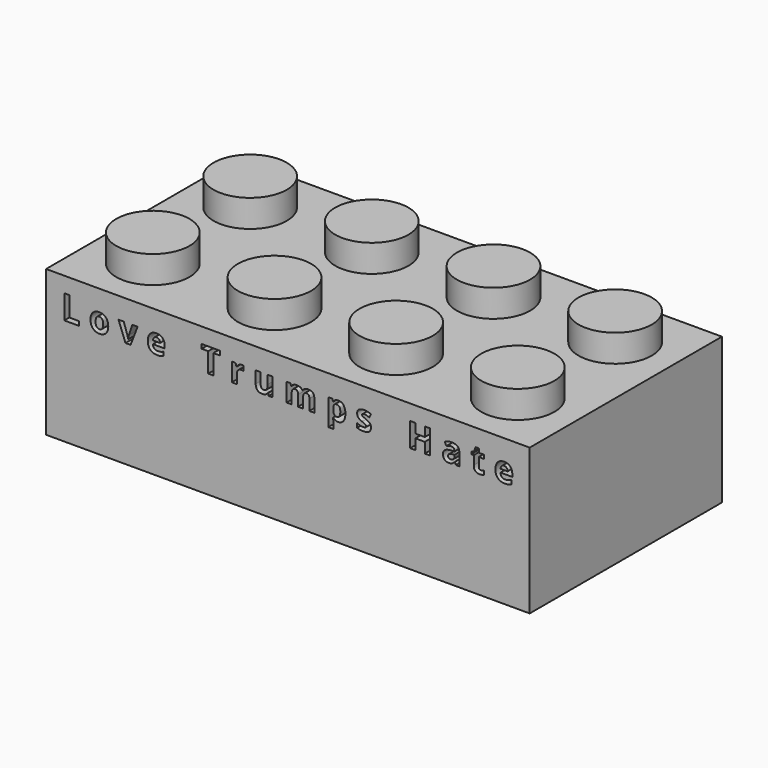
from build123d import *

# Parameters (mm, degrees)
F0_W          = 31.8
F0_H          = 15.8
F1_DEPTH      = 4.8
F2_W          = 29.4
F2_H          = 13.4
F3_DEPTH      = 8.6
F4_R          = 2.409
F5_DEPTH      = 1.8
F6_R          = 1.3
F7_DEPTH      = 1.2
F8_R          = 3.255
F8_R_2        = 2.4
F9_DEPTH      = 8.6
F10_W         = 0.3
F10_H         = 0.6
F11_DEPTH     = 8.6
F12_W         = 0.6
F12_H         = 0.3
F13_DEPTH     = 8.6
F14_W         = 0.8
F14_H         = 3.4696710694
F15_DEPTH     = 6.4
F16_TEXT_SIZE = 2.2075862628
F17_DEPTH     = 1


# Not quite as in the source:
# - Text() gives the source's letters only with a copy of the font that has no kerning and outlines rounded to 1/6400 em; it was checked with that copy


with BuildPart() as f1:
    # F0 (on Top) → F1 (new body, symmetric)
    with BuildSketch(Plane.XY):
        Rectangle(F0_W, F0_H)
    extrude(amount=F1_DEPTH, both=True)

    # F2 (on face) → F3 (cut)
    with BuildSketch(Plane(origin=(0, 0, -4.8), x_dir=(1, 0, 0), z_dir=(0, 0, -1))):
        Rectangle(F2_W, F2_H)
    extrude(amount=-F3_DEPTH, mode=Mode.SUBTRACT)

    # F4 (on face) → F5 (join)
    with BuildSketch(Plane.XY.offset(4.8)):
        with Locations((-12, 4)):
            Circle(F4_R)
        with Locations((-4, 4)):
            Circle(F4_R)
        with Locations((-12, -4)):
            Circle(F4_R)
        with Locations((-4, -4)):
            Circle(F4_R)
        with Locations((4, -4)):
            Circle(F4_R)
        with Locations((12, -4)):
            Circle(F4_R)
        with Locations((4, 4)):
            Circle(F4_R)
        with Locations((12, 4)):
            Circle(F4_R)
    extrude(amount=F5_DEPTH)

    # F6 (on face) → F7 (cut)
    with BuildSketch(Plane(origin=(0, 0, 3.8), x_dir=(1, 0, 0), z_dir=(0, 0, -1))):
        with Locations((-12, 4)):
            Circle(F6_R)
        with Locations((-4, 4)):
            Circle(F6_R)
        with Locations((-4, -4)):
            Circle(F6_R)
        with Locations((-12, -4)):
            Circle(F6_R)
        with Locations((4, -4)):
            Circle(F6_R)
        with Locations((12, -4)):
            Circle(F6_R)
        with Locations((4, 4)):
            Circle(F6_R)
        with Locations((12, 4)):
            Circle(F6_R)
    extrude(amount=-F7_DEPTH, mode=Mode.SUBTRACT)

    # F8 (on face) → F9 (join, through all)
    with BuildSketch(Plane(origin=(0, 0, 3.8), x_dir=(1, 0, 0), z_dir=(0, 0, -1))):
        with Locations((-8, 0)):
            Circle(F8_R)
        with Locations((-8, 0)):
            Circle(F8_R_2, mode=Mode.SUBTRACT)
        Circle(F8_R)
        Circle(F8_R_2, mode=Mode.SUBTRACT)
        with Locations((8, 0)):
            Circle(F8_R)
        with Locations((8, 0)):
            Circle(F8_R_2, mode=Mode.SUBTRACT)
    extrude(amount=F9_DEPTH)

    # F10 (on face) → F11 (join, through all)
    with BuildSketch(Plane(origin=(0, 0, 3.8), x_dir=(1, 0, 0), z_dir=(0, 0, -1))):
        Polygon((-14.7, 4.3), (-14.7, 3.7), (-14.4, 3.7), (-14.4, 4.2064064182), (-14.4, 4.2636040598), (-14.4, 4.3), align=None)
        with Locations((-14.55, -4)):
            Rectangle(F10_W, F10_H)
        with Locations((14.55, -4)):
            Rectangle(F10_W, F10_H)
        with Locations((14.55, 4)):
            Rectangle(F10_W, F10_H)
    extrude(amount=F11_DEPTH)

    # F12 (on face) → F13 (join, through all)
    with BuildSketch(Plane(origin=(0, 0, 3.8), x_dir=(1, 0, 0), z_dir=(0, 0, -1))):
        with Locations((-12, 6.55)):
            Rectangle(F12_W, F12_H)
        with Locations((-4, 6.55)):
            Rectangle(F12_W, F12_H)
        with Locations((4, 6.55)):
            Rectangle(F12_W, F12_H)
        with Locations((12, 6.55)):
            Rectangle(F12_W, F12_H)
        with Locations((-4, -6.55)):
            Rectangle(F12_W, F12_H)
        with Locations((-12, -6.55)):
            Rectangle(F12_W, F12_H)
        with Locations((4, -6.55)):
            Rectangle(F12_W, F12_H)
        with Locations((12, -6.55)):
            Rectangle(F12_W, F12_H)
    extrude(amount=F13_DEPTH)

    # F14 (on face) → F15 (join)
    with BuildSketch(Plane(origin=(0, 0, 3.8), x_dir=(1, 0, 0), z_dir=(0, 0, -1))):
        with Locations((0, 4.9651644653)):
            Rectangle(F14_W, F14_H)
        with Locations((0, -4.9651644653)):
            Rectangle(F14_W, F14_H)
    extrude(amount=F15_DEPTH)

    # F16 (on face) → F17 (cut)
    with BuildSketch(Plane.XZ.offset(7.9)):
        with Locations((-14.9, 2.2105378908)):
            Text('L o v e    T r u m p s    H a t e', F16_TEXT_SIZE, font='Open Sans', font_style=FontStyle.BOLD, text_align=(TextAlign.LEFT, TextAlign.BOTTOM))
    extrude(amount=-F17_DEPTH, mode=Mode.SUBTRACT)


solid = f1.part
